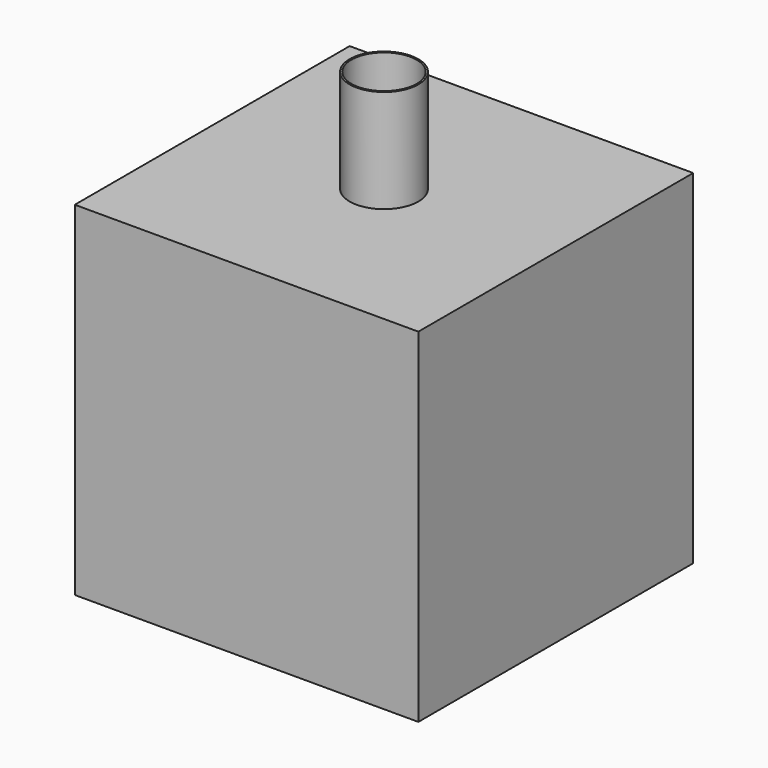
from build123d import *

# Parameters (mm, degrees)
F0_W     = 100
F0_H     = 100
F1_DEPTH = 100
F2_R     = 10
F2_R_2   = 9.5
F3_DEPTH = 30
F4_DEPTH = 100
F5_W     = 98
F5_H     = 98
F5_R     = 9.5
F6_DEPTH = 5


with BuildPart() as f1:
    # F0 (on Top) → F1 (new body)
    with BuildSketch(Plane.XY):
        Rectangle(F0_W, F0_H)
    extrude(amount=-F1_DEPTH)

    # F2 (on Top) → F3 (join)
    with BuildSketch(Plane.XY):
        Circle(F2_R)
        Circle(F2_R_2, mode=Mode.SUBTRACT)
    extrude(amount=F3_DEPTH)

    # F4 (cut, through all): a face of the model
    f4_faces = [f1.faces().sort_by_distance(p)[0] for p in [
        (0, 0, 0),
    ]]
    extrude(f4_faces, amount=-F4_DEPTH, mode=Mode.SUBTRACT)

    # F5 (on face) → F6 (cut)
    with BuildSketch(Plane(origin=(0, 0, -100), x_dir=(1, 0, 0), z_dir=(0, 0, -1))):
        Rectangle(F5_W, F5_H)
        Circle(F5_R, mode=Mode.SUBTRACT)
    extrude(amount=-F6_DEPTH, mode=Mode.SUBTRACT)


solid = f1.part
